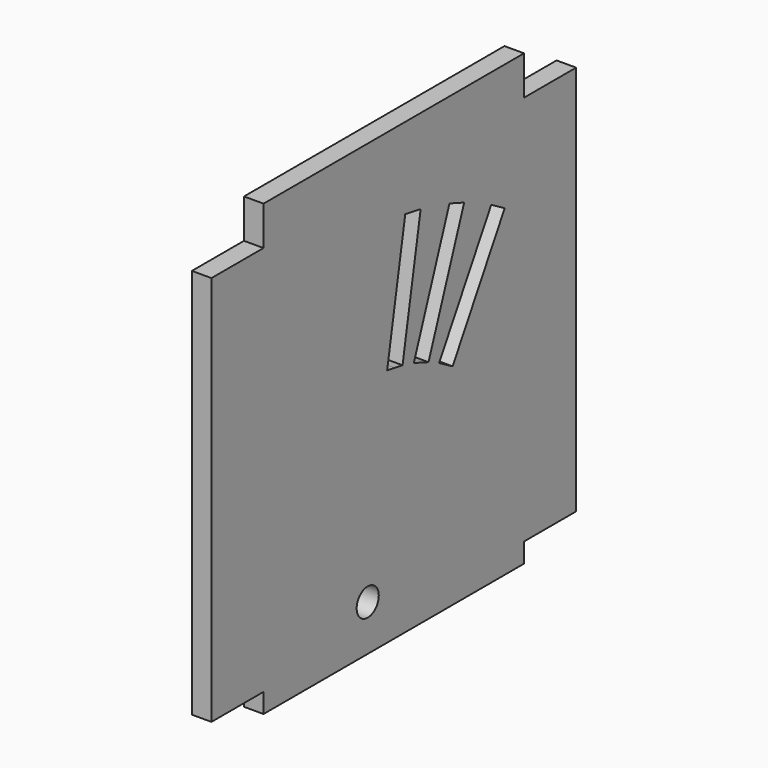
from build123d import *

# Parameters (mm, degrees)
F0_W     = 35
F0_H     = 30
F1_DEPTH = 1.5
F2_W     = 25
F2_H     = 3
F3_DEPTH = 1.5
F4_W     = 25
F4_H     = 1.5
F5_DEPTH = 25
F6_R     = 1.0606601718
F7_DEPTH = 1.501


# Not quite as in the source:
# - a pattern or mirror of a feature is missing from the dataset's text; its kind, count and spacing are read off the source's solid


with BuildPart() as f1:
    # F0 (on Right) → F1 (new body)
    with BuildSketch(Plane.YZ):
        Rectangle(F0_W, F0_H)
    extrude(amount=F1_DEPTH)

    # F2 (on face) → F3 (join)
    with BuildSketch(Plane.YZ.offset(1.5)):
        with Locations((0, 16.5)):
            Rectangle(F2_W, F2_H)
    f3 = extrude(amount=-F3_DEPTH)

    # F3_copies: F3 across plane
    add(f3.mirror(Plane(origin=(0, 0, 0.75), x_dir=(-1, 0, 0), z_dir=(0, 0, -1))))

    # F4 (on face) → F5 (cut)
    with BuildSketch(Plane.YZ.offset(1.5)):
        with Locations((0, -17.25)):
            Rectangle(F4_W, F4_H)
    extrude(amount=-F5_DEPTH, mode=Mode.SUBTRACT)

    # F6 (on face) → F7 (cut, through all)
    with BuildSketch(Plane.YZ.offset(1.5)):
        Polygon((-0.6338831498, 1.9119713717), (0.104722665, 1.7817352384), (0.8433284798, 1.6514991052), (2.5798102564, 11.4995766353), (1.8412044417, 11.6298127685), (1.1025986269, 11.7600489018), align=None)
        with Locations((-2.5, -12.9903810568)):
            Circle(F6_R)
        Polygon((1.9255326843, 1.3615233625), (2.6303021499, 1.105008255), (3.3350716155, 0.8484931475), (6.7552730487, 10.2454193554), (6.0505035831, 10.5019344629), (5.3457341176, 10.7584495704), align=None)
        Polygon((4.3504809472, 0.375), (5, 0), (5.6495190528, -0.375), (10.6495190528, 8.2852540378), (10, 8.6602540378), (9.3504809472, 9.0352540378), align=None)
    extrude(amount=-F7_DEPTH, mode=Mode.SUBTRACT)


solid = f1.part
